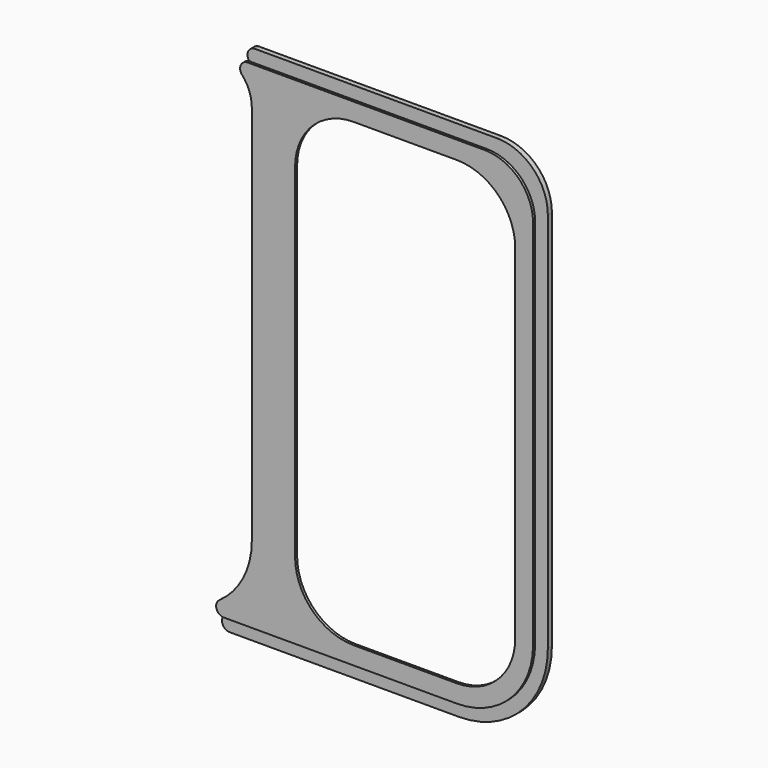
from build123d import *

# Parameters (mm, degrees)
F1_DEPTH = 6
F2_DEPTH = 4
F3_DEPTH = 4
F4_DEPTH = 4


# Not quite as in the source:
# - a feature names something its author has since deleted; it is built from what else it names


with BuildPart() as f1:
    # F0 (on Front) → F1 (new body)
    with BuildSketch(Plane.XZ):
        with BuildLine():
            Line((-100.5, 195), (-100.5, -195))
            Line((-100.5, -195), (-40.5, -195))
            Line((-40.5, -195), (40.5, -195))
            ThreePointArc((40.5, -195), (82.9264068712, -177.4264068712), (100.5, -135))
            Line((100.5, -135), (100.5, 157))
            ThreePointArc((100.5, 157), (89.3700576851, 183.8700576851), (62.5, 195))
            Line((62.5, 195), (-100.5, 195))
        make_face()
        with BuildLine():
            Line((96.5, 157), (96.5, -135))
            ThreePointArc((96.5, -135), (80.0979797464, -174.5979797464), (40.5, -191))
            Line((40.5, -191), (-90.5, -191))
            ThreePointArc((-90.5, -191), (-94.7426406871, -189.2426406871), (-96.5, -185))
            Line((-96.5, -185), (-96.5, 185))
            ThreePointArc((-96.5, 185), (-94.7426406871, 189.2426406871), (-90.5, 191))
            Line((-90.5, 191), (62.5, 191))
            ThreePointArc((62.5, 191), (86.5416305603, 181.0416305603), (96.5, 157))
        make_face(mode=Mode.SUBTRACT)
        with BuildLine():
            ThreePointArc((-142.7480761254, -193.9473684211), (-143.3275959396, -194.3693704052), (-143.8526478713, -194.8574783429))
            ThreePointArc((-143.8526478713, -194.8574783429), (-143.2065526025, -194.9642631589), (-142.552668078, -195))
            Line((-142.552668078, -195), (-100.5, -195))
            Line((-100.5, -195), (-100.5, 195))
            Line((-100.5, 195), (-123.66718427, 195))
            ThreePointArc((-123.66718427, 195), (-123.8241029609, 194.9979476927), (-123.9809143034, 194.9917921748))
            ThreePointArc((-123.9809143034, 194.9917921748), (-123.7745554417, 194.7731997599), (-123.5575071568, 194.5652173913))
            ThreePointArc((-123.5575071568, 194.5652173913), (-113.9097026951, 181.1601405667), (-110.5, 165))
            Line((-110.5, 165), (-110.5, -135))
            ThreePointArc((-110.5, -135), (-119.0889477731, -168.5958727285), (-142.7480761254, -193.9473684211))
        make_face()
        with BuildLine():
            ThreePointArc((-146.0024255254, -184.0909090909), (-148.4365234746, -190.1748385726), (-143.8526478713, -194.8574783429))
            ThreePointArc((-143.8526478713, -194.8574783429), (-143.3275959396, -194.3693704052), (-142.7480761254, -193.9473684211))
            ThreePointArc((-142.7480761254, -193.9473684211), (-119.0889477731, -168.5958727285), (-110.5, -135))
            Line((-110.5, -135), (-110.5, 165))
            ThreePointArc((-110.5, 165), (-113.9097026951, 181.1601405667), (-123.5575071568, 194.5652173913))
            ThreePointArc((-123.5575071568, 194.5652173913), (-123.7745554417, 194.7731997599), (-123.9809143034, 194.9917921748))
            ThreePointArc((-123.9809143034, 194.9917921748), (-129.2065981407, 191.3054053807), (-128.139320225, 185))
            ThreePointArc((-128.139320225, 185), (-122.4748292311, 175.7046626932), (-120.5, 165))
            Line((-120.5, 165), (-120.5, -135))
            ThreePointArc((-120.5, -135), (-127.2559652709, -162.6599487665), (-146.0024255254, -184.0909090909))
        make_face()
        with BuildLine():
            ThreePointArc((40.5, -191), (80.0979797464, -174.5979797464), (96.5, -135))
            Line((96.5, -135), (96.5, 157))
            ThreePointArc((96.5, 157), (86.5416305603, 181.0416305603), (62.5, 191))
            Line((62.5, 191), (-90.5, 191))
            ThreePointArc((-90.5, 191), (-94.7426406871, 189.2426406871), (-96.5, 185))
            Line((-96.5, 185), (-96.5, -185))
            ThreePointArc((-96.5, -185), (-94.7426406871, -189.2426406871), (-90.5, -191))
            Line((-90.5, -191), (40.5, -191))
        make_face()
        with BuildLine():
            Line((86.5, 135), (86.5, -135))
            ThreePointArc((86.5, -135), (73.0269119346, -167.5269119346), (40.5, -181))
            Line((40.5, -181), (-40.5, -181))
            ThreePointArc((-40.5, -181), (-73.0269119346, -167.5269119346), (-86.5, -135))
            Line((-86.5, -135), (-86.5, 135))
            ThreePointArc((-86.5, 135), (-73.0269119346, 167.5269119346), (-40.5, 181))
            Line((-40.5, 181), (40.5, 181))
            ThreePointArc((40.5, 181), (73.0269119346, 167.5269119346), (86.5, 135))
        make_face(mode=Mode.SUBTRACT)
    extrude(amount=F1_DEPTH)

    # F0 (on Front) → F2 (join)
    with BuildSketch(Plane.XZ):
        with BuildLine():
            Line((-110.5, -205), (40.5, -205))
            ThreePointArc((40.5, -205), (89.9974746831, -184.4974746831), (110.5, -135))
            Line((110.5, -135), (110.5, 165))
            ThreePointArc((110.5, 165), (98.7842712475, 193.2842712475), (70.5, 205))
            Line((70.5, 205), (-110.5, 205))
            Line((-110.5, 205), (-119.5161332303, 205))
            ThreePointArc((-119.5161332303, 205), (-124.9956061498, 201.4444583295), (-123.9809143034, 194.9917921748))
            ThreePointArc((-123.9809143034, 194.9917921748), (-123.8241029609, 194.9979476927), (-123.66718427, 195))
            Line((-123.66718427, 195), (-100.5, 195))
            Line((-100.5, 195), (62.5, 195))
            ThreePointArc((62.5, 195), (89.3700576851, 183.8700576851), (100.5, 157))
            Line((100.5, 157), (100.5, -135))
            ThreePointArc((100.5, -135), (82.9264068712, -177.4264068712), (40.5, -195))
            Line((40.5, -195), (-40.5, -195))
            Line((-40.5, -195), (-100.5, -195))
            Line((-100.5, -195), (-142.552668078, -195))
            ThreePointArc((-142.552668078, -195), (-143.2065526025, -194.9642631589), (-143.8526478713, -194.8574783429))
            ThreePointArc((-143.8526478713, -194.8574783429), (-145.0283155871, -201.3606005652), (-139.5121969362, -205))
            Line((-139.5121969362, -205), (-110.5, -205))
        make_face()
    extrude(amount=F2_DEPTH)

    # F0 (on Front) → F3 (cut)
    with BuildSketch(Plane.XZ):
        with BuildLine():
            ThreePointArc((-146.0024255254, -184.0909090909), (-148.4365234746, -190.1748385726), (-143.8526478713, -194.8574783429))
            ThreePointArc((-143.8526478713, -194.8574783429), (-143.3275959396, -194.3693704052), (-142.7480761254, -193.9473684211))
            ThreePointArc((-142.7480761254, -193.9473684211), (-119.0889477731, -168.5958727285), (-110.5, -135))
            Line((-110.5, -135), (-110.5, 165))
            ThreePointArc((-110.5, 165), (-113.9097026951, 181.1601405667), (-123.5575071568, 194.5652173913))
            ThreePointArc((-123.5575071568, 194.5652173913), (-123.7745554417, 194.7731997599), (-123.9809143034, 194.9917921748))
            ThreePointArc((-123.9809143034, 194.9917921748), (-129.2065981407, 191.3054053807), (-128.139320225, 185))
            ThreePointArc((-128.139320225, 185), (-122.4748292311, 175.7046626932), (-120.5, 165))
            Line((-120.5, 165), (-120.5, -135))
            ThreePointArc((-120.5, -135), (-127.2559652709, -162.6599487665), (-146.0024255254, -184.0909090909))
        make_face()
    extrude(amount=F3_DEPTH, mode=Mode.SUBTRACT)

    # F0 (on Front) → F4 (cut)
    with BuildSketch(Plane.XZ):
        with BuildLine():
            ThreePointArc((40.5, -191), (80.0979797464, -174.5979797464), (96.5, -135))
            Line((96.5, -135), (96.5, 157))
            ThreePointArc((96.5, 157), (86.5416305603, 181.0416305603), (62.5, 191))
            Line((62.5, 191), (-90.5, 191))
            ThreePointArc((-90.5, 191), (-94.7426406871, 189.2426406871), (-96.5, 185))
            Line((-96.5, 185), (-96.5, -185))
            ThreePointArc((-96.5, -185), (-94.7426406871, -189.2426406871), (-90.5, -191))
            Line((-90.5, -191), (40.5, -191))
        make_face()
        with BuildLine():
            Line((86.5, 135), (86.5, -135))
            ThreePointArc((86.5, -135), (73.0269119346, -167.5269119346), (40.5, -181))
            Line((40.5, -181), (-40.5, -181))
            ThreePointArc((-40.5, -181), (-73.0269119346, -167.5269119346), (-86.5, -135))
            Line((-86.5, -135), (-86.5, 135))
            ThreePointArc((-86.5, 135), (-73.0269119346, 167.5269119346), (-40.5, 181))
            Line((-40.5, 181), (40.5, 181))
            ThreePointArc((40.5, 181), (73.0269119346, 167.5269119346), (86.5, 135))
        make_face(mode=Mode.SUBTRACT)
    extrude(amount=F4_DEPTH, mode=Mode.SUBTRACT)


solid = f1.part
